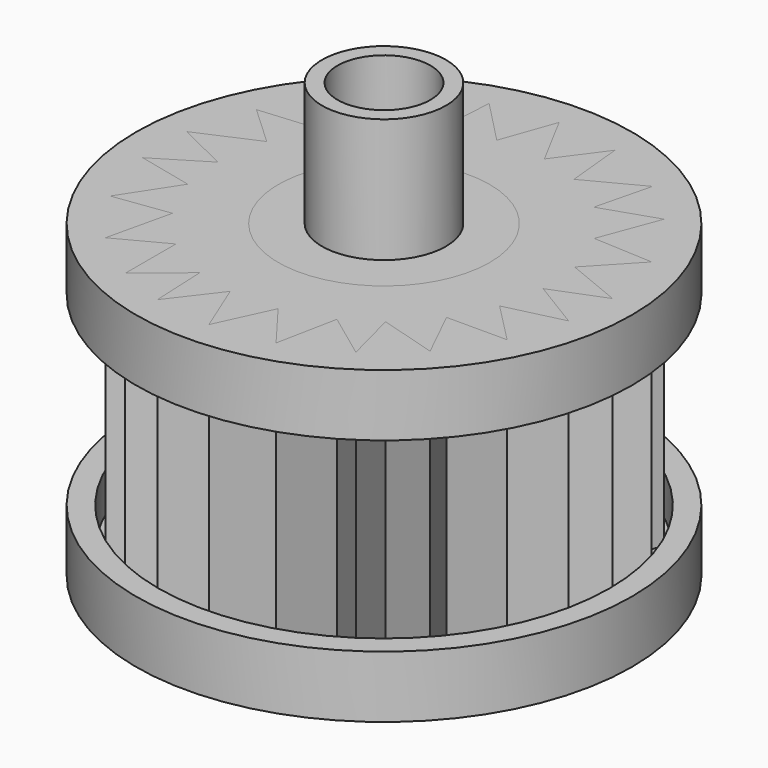
from build123d import *

# Parameters (mm, degrees)
F0_R     = 6.35
F0_R_2   = 4.7625
F1_DEPTH = 12.7
F2_R     = 25.4
F3_DEPTH = 6.35
F4_T     = 2.286
F6_R     = 25.4
F7_DEPTH = 6.35
F8_T     = -2.286
F9_R     = 10.8324762704


# Not quite as in the source:
# - a shell that OpenCascade refuses in one call is made with other operations: the cavity is built on its own and cut out


with BuildPart() as f1:
    # F0 (on Top) → F1 (new body)
    with BuildSketch(Plane.XY):
        Circle(F0_R)
        Circle(F0_R_2, mode=Mode.SUBTRACT)
    extrude(amount=F1_DEPTH)

    # F2 (on Top) → F3 (join)
    with BuildSketch(Plane.XY):
        Circle(F2_R)
    extrude(amount=-F3_DEPTH)

    # F4: shell of thickness 2.286, made by hand


with BuildPart() as f4_core1:
    # F4_t2: copy of F1
    add(f1.part)

    # the walls: a layer under each face that stays
    f4_faces = [f4_core1.faces().sort_by_distance(p)[0] for p in [
        (-25.4, 0, -3.175),
        (-16.9333333333, -16.9333333333, 0),
        (-6.35, 0, 6.35),
        (-4.2333333333, -4.2333333333, 12.7),
        (-4.7625, 0, 6.35),
        (0, 0, 0),
    ]]
    thicken(f4_faces, amount=-F4_T, mode=Mode.SUBTRACT)

    # F4_s3 → F4_t4 (revolve, cut)
    with BuildSketch(Plane.XZ):
        Polygon((6.37286, 0.02286), (6.35, -2.286), (4.064, -2.286), (4.064, 0), align=None)
    revolve(axis=Axis((0, 0, 0), (0, 0, 1)), mode=Mode.SUBTRACT)

    # F4_s5 → F4_t6 (revolve, cut)
    with BuildSketch(Plane.XZ):
        Polygon((4.73964, 0.02286), (7.0485, 0), (7.0485, -2.286), (4.7625, -2.286), align=None)
    revolve(axis=Axis((0, 0, 0), (0, 0, 1)), mode=Mode.SUBTRACT)


with BuildPart() as f1_1:
    add(f1.part)

    # what is left inside the walls is the cavity
    f4_cavity = [f4_core1.part.solids().sort_by_distance(p)[0] for p in [
        (0, -7.704667, -2.30886),
    ]]
    add(f4_cavity, mode=Mode.SUBTRACT)


with BuildPart() as f7:
    # F6 (on offset) → F7 (new body)
    with BuildSketch(Plane.XY.offset(-31.75)):
        Circle(F6_R)
    extrude(amount=F7_DEPTH)

    # F8
    f8_openings = [f7.faces().sort_by_distance(p)[0] for p in [
        (0, 0, -25.4),
    ]]
    offset(amount=F8_T, openings=f8_openings)


with BuildPart() as f11:
    # F11: sweep along a path in F10
    with BuildLine(Plane.YZ) as f11_path:
        Line((0, 0), (0, -31.5147303045))
    # F9 (on Top) → F11 (sweep)
    with BuildSketch(Plane.XY):
        Polygon((-22.2801696853, 2.5754143982), (-17.0194395337, 0), (-22.2047725652, -3.1601892119), (-16.5178161114, -4.4880653732), (-20.0906647852, -9.9701509023), (-14.3254104125, -9.1893383088), (-15.8624105906, -15.8563126477), (-10.7827289936, -13.167918495), (-10.7827289936, -19.6665064508), (-6.1837424961, -15.8563126477), (-5.9169946662, -21.6339523585), (-2.2652936168, -16.8680101633), (0, -22.4285247069), (2.6029271509, -16.8192179452), (6.1861512021, -21.558530883), (7.4289074138, -15.3125000139), (12.1825904339, -18.8314420809), (10.7273710707, -13.2130553602), (16.7018596911, -14.9695224836), (14.0682479763, -9.5783986615), (20.2803599477, -9.5783986615), (16.1477248117, -5.3770164073), (22.0774019915, -3.9531053404), (16.99756164, -0.8626820586), (22.3925396791, 1.2699949796), (16.6237094694, 3.648781374), (20.8843409163, 8.1782042663), (14.7502192053, 8.4907217263), (17.0355213321, 14.588685118), (11.3350188011, 12.6956162047), (12.7622102664, 18.4435546911), (7.0890507934, 15.4727722432), (6.4961991134, 21.4671404152), (3.0343190109, 16.7467677532), (0, 22.4285247069), (-1.9673980921, 16.9053443262), (-6.4182103819, 21.4905862186), (-6.8137495325, 15.595965483), (-12.4052478598, 18.6855170136), (-10.9380790438, 13.0391621231), (-16.9691750647, 14.3013333161), (-14.0740074147, 9.5699340295), (-20.2957504461, 9.0299506542), (-16.1967538501, 5.2274742237), align=None)
        Circle(F9_R, mode=Mode.SUBTRACT)
    sweep(path=f11_path.line)


solid = Compound([f1_1.part, f7.part, f11.part])
